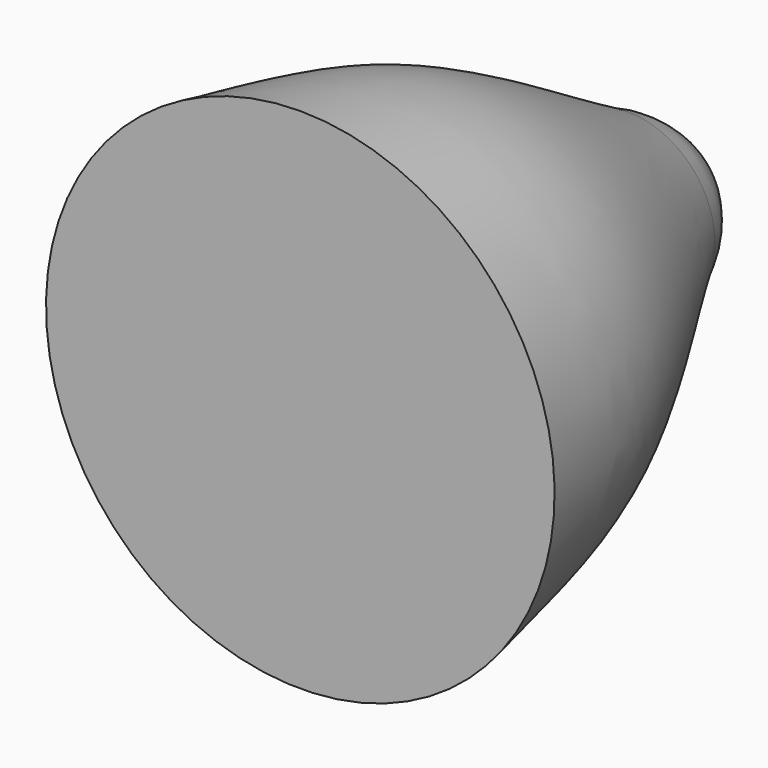
from build123d import *


# Not quite as in the source:
# - a feature of the source that left no trace in its solid (it failed there, or was rolled back) is left out
# - the program builds the solid bodies; features that only make, move or delete a surface that nothing else refers to are left out


with BuildPart() as f1:
    # F0 (on Right) → F1 (revolve)
    with BuildSketch(Plane.YZ):
        with BuildLine():
            ThreePointArc((69.6175396442, 0), (65.2988703753, 7.4584587089), (58.2477152348, 12.4143362045))
            add(Edge.make_bspline(
                [(58.2477152348, 12.4143362045), (47.9688050987, 18.1678310384), (28.4475695168, 31.6564253526), (9.1404896716, 34.1858867887), (0, 36.1830964684)],
                knots=[0, 0, 0, 0, 0.5270994017, 1, 1, 1, 1], degree=3))
            Line((0, 36.1830964684), (0, 0))
            Line((0, 0), (69.6175396442, 0))
        make_face()
    revolve(axis=Axis((0, 34.8087698221, 0), (0, 1, 0)))


solid = f1.part
